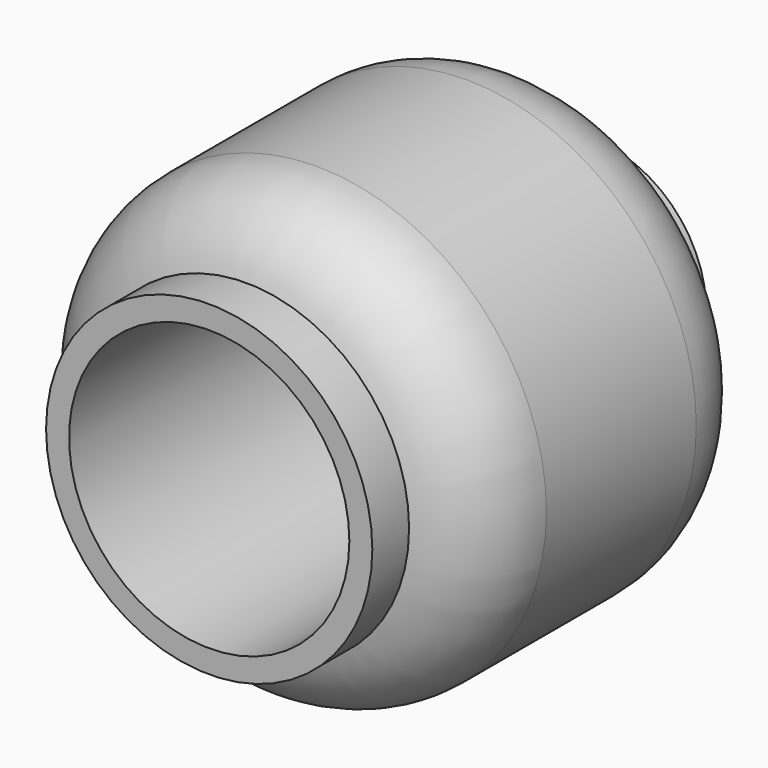
from build123d import *

# Parameters (mm, degrees)
F0_R     = 3.55
F0_R_2   = 3.05
F1_DEPTH = 1
F2_R     = 5
F3_DEPTH = 8
F5_R     = 2.5
F5_R_2   = 2
F6_DEPTH = 1.4
F8_DEPTH = 5


# Not quite as in the source:
# - a fillet or chamfer that OpenCascade refuses, or shapes differently, is made with other operations: its cross-section is extruded or revolved along the edge and cut away or added


with BuildPart() as f1:
    # F0 (on Front) → F1 (new body)
    with BuildSketch(Plane.XZ):
        Circle(F0_R)
        Circle(F0_R_2, mode=Mode.SUBTRACT)
    extrude(amount=F1_DEPTH)

    # F2 (on Front) → F3 (join)
    with BuildSketch(Plane.XZ):
        Circle(F2_R)
    extrude(amount=-F3_DEPTH)

    # F5 (on face) → F6 (join)
    with BuildSketch(Plane(origin=(0, 8, 0), x_dir=(-1, 0, 0), z_dir=(0, 1, 0))):
        Circle(F5_R)
        Circle(F5_R_2, mode=Mode.SUBTRACT)
    extrude(amount=F6_DEPTH)

    # F7: fillet of radius 2 on 2 edges, made by hand

    # F7_s1 → F7_t2 (revolve, cut)
    with BuildSketch(Plane.XY):
        with BuildLine():
            ThreePointArc((5, 6), (4.4142135624, 7.4142135624), (3, 8))
            Line((3, 8), (5, 8))
            Line((5, 8), (5, 6))
        make_face()
    revolve(axis=Axis((0, 8, 0), (0, -1, 0)), mode=Mode.SUBTRACT)

    # F7_s3 → F7_t4 (revolve, cut)
    with BuildSketch(Plane.XY):
        with BuildLine():
            ThreePointArc((5, 1.9228884523), (4.5968719423, 0.7187289944), (3.55, 0))
            Line((3.55, 0), (5, 0))
            Line((5, 0), (5, 1.9228884523))
        make_face()
    revolve(axis=Axis((0, 0, 0), (0, -1, 0)), mode=Mode.SUBTRACT)

    # F8 (cut): a face of the model
    f8_faces = [f1.faces().sort_by_distance(p)[0] for p in [
        (0, 0, 0),
    ]]
    extrude(f8_faces, amount=-F8_DEPTH, mode=Mode.SUBTRACT)


solid = f1.part
